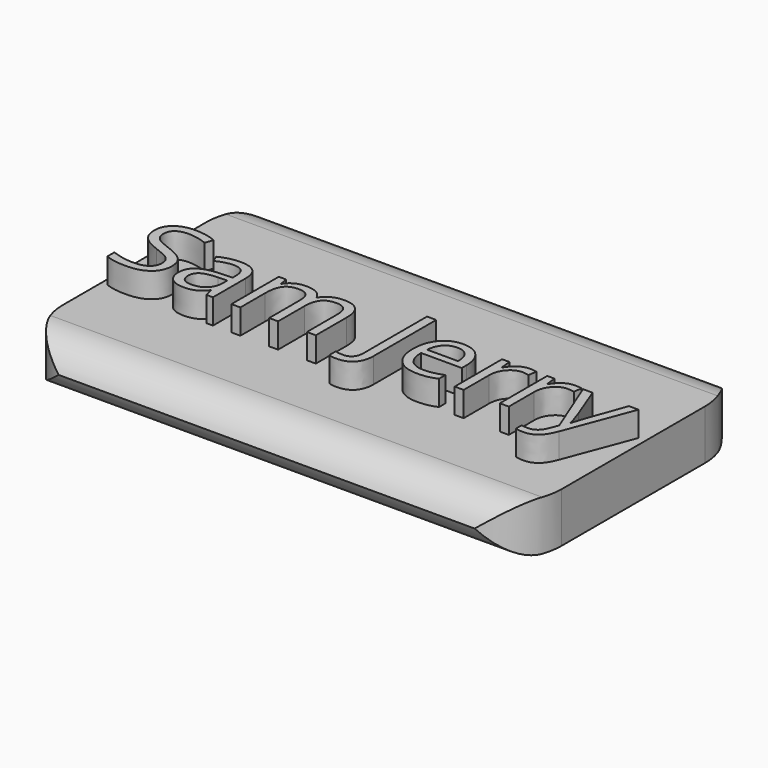
from build123d import *

# Parameters (mm, degrees)
F0_W         = 63.5
F0_H         = 38.1
F1_DEPTH     = 6.35
F2_TEXT_SIZE = 14.0876317249
F3_DEPTH     = 3.175
F4_R         = 7.62
F5_T1_DEPTH  = 73.66


# Not quite as in the source:
# - a fillet or chamfer that OpenCascade refuses, or shapes differently, is made with other operations: its cross-section is extruded or revolved along the edge and cut away or added
# - Text() gives the source's letters only with a copy of the font that has no kerning and outlines rounded to 1/6400 em; it was checked with that copy


with BuildPart() as f1:
    # F0 (on Top) → F1 (new body)
    with BuildSketch(Plane.XY):
        with Locations((31.75, 19.05)):
            Rectangle(F0_W, F0_H)
    extrude(amount=F1_DEPTH)

    # F2 (on face) → F3 (join)
    with BuildSketch(Plane.XY.offset(6.35)):
        with Locations((0, 13.4815445925)):
            Text('Sam Jerry', F2_TEXT_SIZE, font='Open Sans', text_align=(TextAlign.LEFT, TextAlign.BOTTOM))
    extrude(amount=F3_DEPTH)

    # F4
    f4_edges = [f1.edges().sort_by_distance(p)[0] for p in [
        (63.5, 38.1, 3.175),
        (63.5, 0, 3.175),
        (0, 38.1, 3.175),
        (0, 0, 3.175),
    ]]
    fillet(f4_edges, radius=F4_R)

    # F5: fillet of radius 5.08 on 8 edges, made by hand

    # F5_s2 → F5_t1 (cut)
    with BuildSketch(Plane.YZ.offset(-5.08)):
        with BuildLine():
            ThreePointArc((33.02, 0), (36.6121024484, 1.4878975516), (38.1, 5.08))
            Line((38.1, 5.08), (38.1, 0))
            Line((38.1, 0), (33.02, 0))
        make_face()
        with BuildLine():
            ThreePointArc((33.02, 6.35), (36.6121024484, 4.8621024484), (38.1, 1.27))
            Line((38.1, 1.27), (38.1, 6.35))
            Line((38.1, 6.35), (33.02, 6.35))
        make_face()
        with BuildLine():
            ThreePointArc((5.08, 0), (1.4878975516, 1.4878975516), (0, 5.08))
            Line((0, 5.08), (0, 0))
            Line((0, 0), (5.08, 0))
        make_face()
        with BuildLine():
            ThreePointArc((5.08, 6.35), (1.4878975516, 4.8621024484), (0, 1.27))
            Line((0, 1.27), (0, 6.35))
            Line((0, 6.35), (5.08, 6.35))
        make_face()
    extrude(amount=F5_T1_DEPTH, mode=Mode.SUBTRACT)


solid = f1.part
